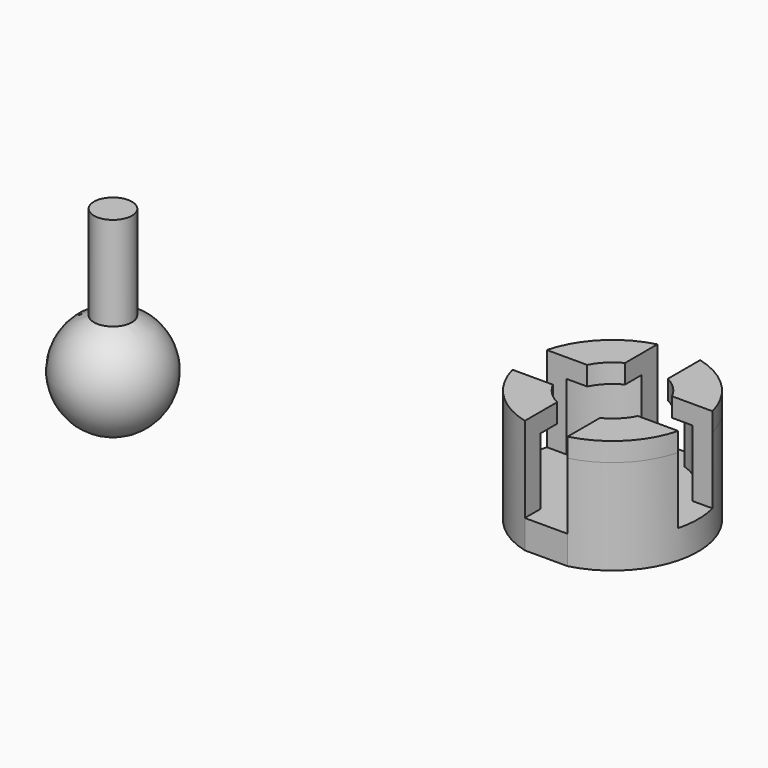
from build123d import *

# Parameters (mm, degrees)
F3_R      = 2
F4_DEPTH  = 15
F6_DEPTH  = 3
F8_DEPTH  = 7
F10_DEPTH = 2


with BuildPart() as f2:
    # F1 (on Top) → F2 (revolve)
    with BuildSketch(Plane.XY):
        with BuildLine():
            Line((-48.6443726491, -10.3812959576), (-48.6443726491, 0.6187040424))
            ThreePointArc((-48.6443726491, 0.6187040424), (-54.1443726491, -4.8812959576), (-48.6443726491, -10.3812959576))
        make_face()
    revolve(axis=Axis((-48.6443726491, -4.8812959576, 0), (0, -1, 0)))

    # F3 (on Top) → F4 (join)
    with BuildSketch(Plane.XY):
        with Locations((-48.6443726491, -4.8812959576)):
            Circle(F3_R)
    extrude(amount=F4_DEPTH)


with BuildPart() as f6:
    # F5 (on Top) + F0 (on Top) → F6 (new body)
    with BuildSketch(Plane.XY):
        with BuildLine():
            ThreePointArc((-4.4651427749, 2.25), (-3.5355339059, 3.5355339059), (-2.25, 4.4651427749))
            Line((-2.25, 4.4651427749), (-2.25, 8.714212529))
            ThreePointArc((-2.25, 8.714212529), (-6.3639610307, 6.3639610307), (-8.714212529, 2.25))
            Line((-8.714212529, 2.25), (-4.4651427749, 2.25))
        make_face()
        with BuildLine():
            ThreePointArc((-2.25, -4.4651427749), (-3.5355339059, -3.5355339059), (-4.4651427749, -2.25))
            Line((-4.4651427749, -2.25), (-8.714212529, -2.25))
            ThreePointArc((-8.714212529, -2.25), (-6.3639610307, -6.3639610307), (-2.25, -8.714212529))
            Line((-2.25, -8.714212529), (-2.25, -4.4651427749))
        make_face()
        with BuildLine():
            ThreePointArc((2.25, -8.714212529), (6.3639610307, -6.3639610307), (8.714212529, -2.25))
            Line((8.714212529, -2.25), (4.4651427749, -2.25))
            ThreePointArc((4.4651427749, -2.25), (3.5355339059, -3.5355339059), (2.25, -4.4651427749))
            Line((2.25, -4.4651427749), (2.25, -8.714212529))
        make_face()
        with BuildLine():
            Line((-2.25, 8.714212529), (-2.25, 4.4651427749))
            ThreePointArc((-2.25, 4.4651427749), (-3.5355339059, 3.5355339059), (-4.4651427749, 2.25))
            ThreePointArc((-4.4651427749, 2.25), (-5, 0), (-4.4651427749, -2.25))
            ThreePointArc((-4.4651427749, -2.25), (-3.5355339059, -3.5355339059), (-2.25, -4.4651427749))
            Line((-2.25, -4.4651427749), (-2.25, -8.714212529))
            Line((-2.25, -8.714212529), (2.25, -8.714212529))
            Line((2.25, -8.714212529), (2.25, -4.4651427749))
            ThreePointArc((2.25, -4.4651427749), (3.5355339059, -3.5355339059), (4.4651427749, -2.25))
            ThreePointArc((4.4651427749, -2.25), (5, 0), (4.4651427749, 2.25))
            ThreePointArc((4.4651427749, 2.25), (3.5355339059, 3.5355339059), (2.25, 4.4651427749))
            Line((2.25, 4.4651427749), (2.25, 8.714212529))
            Line((2.25, 8.714212529), (-2.25, 8.714212529))
        make_face()
    with BuildSketch(Plane.XY):
        with BuildLine():
            ThreePointArc((-4.4651427749, -2.25), (-5, 0), (-4.4651427749, 2.25))
            Line((-4.4651427749, 2.25), (-8.714212529, 2.25))
            ThreePointArc((-8.714212529, 2.25), (-9, 0), (-8.714212529, -2.25))
            Line((-8.714212529, -2.25), (-4.4651427749, -2.25))
        make_face()
        with BuildLine():
            ThreePointArc((8.714212529, -2.25), (9, 0), (8.714212529, 2.25))
            Line((8.714212529, 2.25), (4.4651427749, 2.25))
            ThreePointArc((4.4651427749, 2.25), (5, 0), (4.4651427749, -2.25))
            Line((4.4651427749, -2.25), (8.714212529, -2.25))
        make_face()
        with BuildLine():
            ThreePointArc((8.714212529, 2.25), (6.3639610307, 6.3639610307), (2.25, 8.714212529))
            Line((2.25, 8.714212529), (2.25, 4.4651427749))
            ThreePointArc((2.25, 4.4651427749), (3.5355339059, 3.5355339059), (4.4651427749, 2.25))
            Line((4.4651427749, 2.25), (8.714212529, 2.25))
        make_face()
    extrude(amount=F6_DEPTH)

    # F7 (on face) → F8 (join)
    with BuildSketch(Plane.XY.offset(3)):
        with BuildLine():
            ThreePointArc((-6.6285367918, 2.25), (-4.9497474683, 4.9497474683), (-2.25, 6.6285367918))
            Line((-2.25, 6.6285367918), (-2.25, 8.714212529))
            ThreePointArc((-2.25, 8.714212529), (-6.3639610307, 6.3639610307), (-8.714212529, 2.25))
            Line((-8.714212529, 2.25), (-6.6285367918, 2.25))
        make_face()
        with BuildLine():
            ThreePointArc((8.714212529, 2.25), (6.3639610307, 6.3639610307), (2.25, 8.714212529))
            Line((2.25, 8.714212529), (2.25, 6.6285367918))
            ThreePointArc((2.25, 6.6285367918), (4.9497474683, 4.9497474683), (6.6285367918, 2.25))
            Line((6.6285367918, 2.25), (8.714212529, 2.25))
        make_face()
        with BuildLine():
            ThreePointArc((2.25, -8.714212529), (6.3639610307, -6.3639610307), (8.714212529, -2.25))
            Line((8.714212529, -2.25), (6.6285367918, -2.25))
            ThreePointArc((6.6285367918, -2.25), (4.9497474683, -4.9497474683), (2.25, -6.6285367918))
            Line((2.25, -6.6285367918), (2.25, -8.714212529))
        make_face()
        with BuildLine():
            ThreePointArc((-2.25, -6.6285367918), (-4.9497474683, -4.9497474683), (-6.6285367918, -2.25))
            Line((-6.6285367918, -2.25), (-8.714212529, -2.25))
            ThreePointArc((-8.714212529, -2.25), (-6.3639610307, -6.3639610307), (-2.25, -8.714212529))
            Line((-2.25, -8.714212529), (-2.25, -6.6285367918))
        make_face()
    extrude(amount=F8_DEPTH)

    # F9 (on face) + F8_face (on face) → F10 (join)
    with BuildSketch(Plane.XY.offset(10)):
        with BuildLine():
            ThreePointArc((-6.6285367918, 2.25), (-4.9497474683, 4.9497474683), (-2.25, 6.6285367918))
            Line((-2.25, 6.6285367918), (-2.25, 8.714212529))
            ThreePointArc((-2.25, 8.714212529), (-6.3639610307, 6.3639610307), (-8.714212529, 2.25))
            Line((-8.714212529, 2.25), (-6.6285367918, 2.25))
        make_face()
        with BuildLine():
            ThreePointArc((-4.4651427749, 2.25), (-3.5355339059, 3.5355339059), (-2.25, 4.4651427749))
            Line((-2.25, 4.4651427749), (-2.25, 6.6285367918))
            ThreePointArc((-2.25, 6.6285367918), (-4.9497474683, 4.9497474683), (-6.6285367918, 2.25))
            Line((-6.6285367918, 2.25), (-4.4651427749, 2.25))
        make_face()
        with BuildLine():
            ThreePointArc((6.6285367918, 2.25), (4.9497474683, 4.9497474683), (2.25, 6.6285367918))
            Line((2.25, 6.6285367918), (2.25, 4.4651427749))
            ThreePointArc((2.25, 4.4651427749), (3.5355339059, 3.5355339059), (4.4651427749, 2.25))
            Line((4.4651427749, 2.25), (6.6285367918, 2.25))
        make_face()
        with BuildLine():
            Line((2.25, -4.4651427749), (2.25, -6.6285367918))
            ThreePointArc((2.25, -6.6285367918), (4.9497474683, -4.9497474683), (6.6285367918, -2.25))
            Line((6.6285367918, -2.25), (4.4651427749, -2.25))
            ThreePointArc((4.4651427749, -2.25), (3.5355339059, -3.5355339059), (2.25, -4.4651427749))
        make_face()
        with BuildLine():
            ThreePointArc((-2.25, -4.4651427749), (-3.5355339059, -3.5355339059), (-4.4651427749, -2.25))
            Line((-4.4651427749, -2.25), (-6.6285367918, -2.25))
            ThreePointArc((-6.6285367918, -2.25), (-4.9497474683, -4.9497474683), (-2.25, -6.6285367918))
            Line((-2.25, -6.6285367918), (-2.25, -4.4651427749))
        make_face()
    with BuildSketch(Plane(origin=(-5.466060035, 5.466060035, 10), x_dir=(1, 0, 0), z_dir=(0, 0, 1))):
        with BuildLine():
            Line((12.0945968267, -3.216060035), (14.1802725639, -3.216060035))
            ThreePointArc((14.1802725639, -3.216060035), (11.8300210656, 0.8979009957), (7.716060035, 3.248152494))
            Line((7.716060035, 3.248152494), (7.716060035, 1.1624767568))
            ThreePointArc((7.716060035, 1.1624767568), (10.4158075033, -0.5163125667), (12.0945968267, -3.216060035))
        make_face()
        with BuildLine():
            ThreePointArc((12.0945968267, -7.716060035), (10.4158075033, -10.4158075033), (7.716060035, -12.0945968267))
            Line((7.716060035, -12.0945968267), (7.716060035, -14.1802725639))
            ThreePointArc((7.716060035, -14.1802725639), (11.8300210656, -11.8300210656), (14.1802725639, -7.716060035))
            Line((14.1802725639, -7.716060035), (12.0945968267, -7.716060035))
        make_face()
        with BuildLine():
            Line((3.216060035, -14.1802725639), (3.216060035, -12.0945968267))
            ThreePointArc((3.216060035, -12.0945968267), (0.5163125667, -10.4158075033), (-1.1624767568, -7.716060035))
            Line((-1.1624767568, -7.716060035), (-3.248152494, -7.716060035))
            ThreePointArc((-3.248152494, -7.716060035), (-0.8979009957, -11.8300210656), (3.216060035, -14.1802725639))
        make_face()
    extrude(amount=F10_DEPTH)


solid = Compound([f2.part, f6.part])
